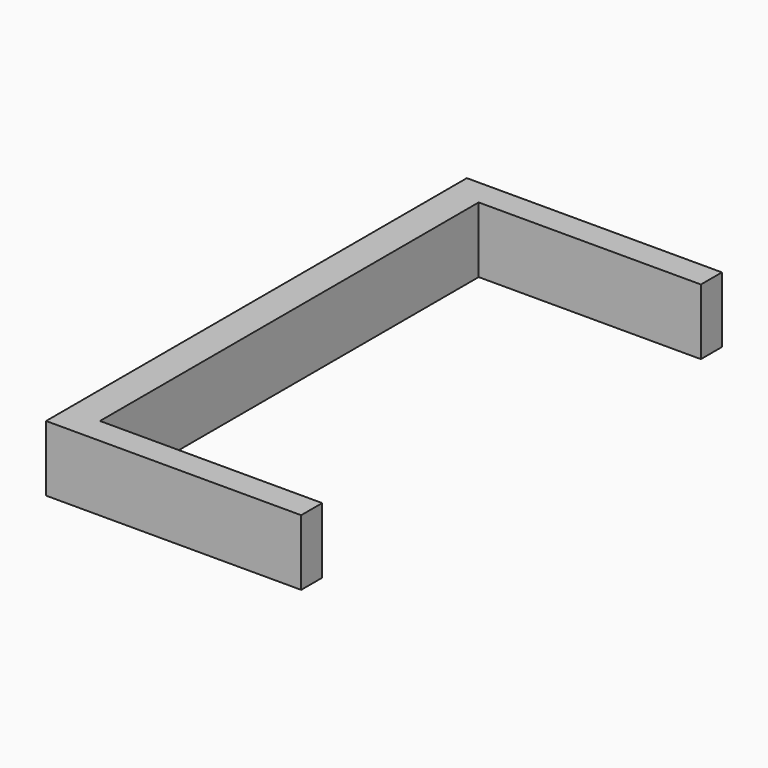
from build123d import *

# Parameters (mm, degrees)
F5_W     = 101.6
F5_H     = 12.7
F6_DEPTH = 6.35
F7_W     = 5.08
F7_H     = 12.7
F8_DEPTH = 42.926


# Not quite as in the source:
# - a feature of the source that left no trace in its solid (it failed there, or was rolled back) is left out


with BuildPart() as f6:
    # F5 (on Right) → F6 (new body)
    with BuildSketch(Plane.YZ):
        with Locations((-2.5232887447, 14.3209207639)):
            Rectangle(F5_W, F5_H)
    extrude(amount=F6_DEPTH)

    # F7 (on face) → F8 (join)
    with BuildSketch(Plane.YZ.offset(6.35)):
        with Locations((-50.7832887447, 14.3209207639)):
            Rectangle(F7_W, F7_H)
        with Locations((45.7367112553, 14.3209207639)):
            Rectangle(F7_W, F7_H)
    extrude(amount=F8_DEPTH)


solid = f6.part
